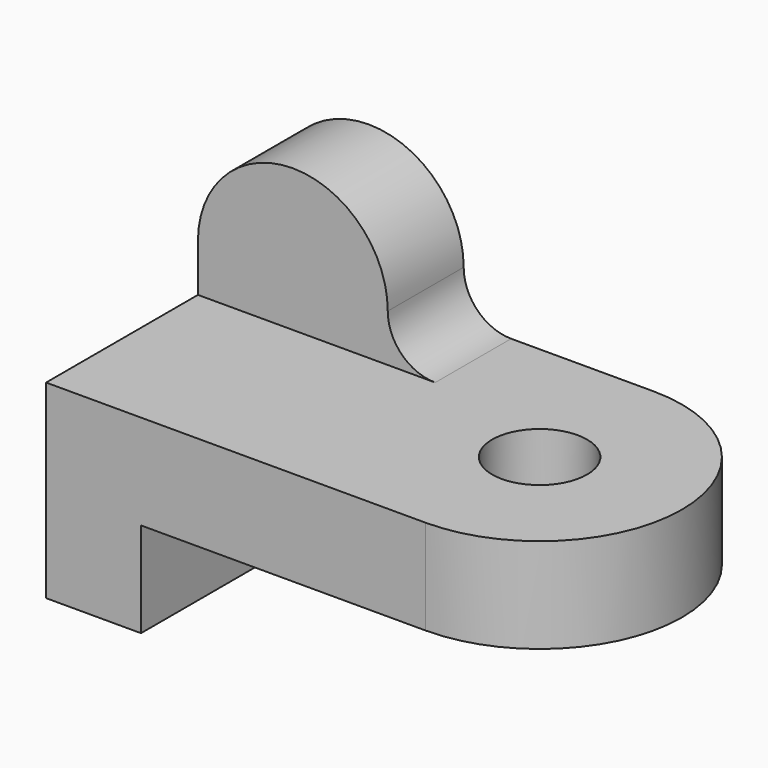
from build123d import *

# Parameters (mm, degrees)
F0_R     = 6.35
F0_W     = 12.7
F0_H     = 25.4
F0_H_2   = 12.7
F1_DEPTH = 12.7
F2_DEPTH = 12.7
F3_DEPTH = 19.05
F4_DEPTH = 12.7
F6_DEPTH = 12.7
F7_R     = 6.34999


# Not quite as in the source:
# - a fillet or chamfer is up to 0.001 mm smaller than in the source, because OpenCascade refuses the exact size


with BuildPart() as f1:
    # F0 (on Top) → F1 (new body)
    with BuildSketch(Plane.XY):
        with BuildLine():
            ThreePointArc((0, -17.2810847643), (19.05, 1.7689152357), (0, 20.8189152357))
            Line((0, 20.8189152357), (-25.4, 20.8189152357))
            Line((-25.4, 20.8189152357), (-25.4, 8.1189152357))
            Line((-25.4, 8.1189152357), (-38.1, 8.1189152357))
            Line((-38.1, 8.1189152357), (-38.1, -17.2810847643))
            Line((-38.1, -17.2810847643), (0, -17.2810847643))
        make_face()
        with Locations((0, 1.7689152357)):
            Circle(F0_R, mode=Mode.SUBTRACT)
        with Locations((-44.45, -4.5810847643)):
            Rectangle(F0_W, F0_H)
        with Locations((-44.45, 14.4689152357)):
            Rectangle(F0_W, F0_H_2)
        with Locations((-31.75, 14.4689152357)):
            Rectangle(F0_W, F0_H_2)
    extrude(amount=F1_DEPTH)

    # F0 (on Top) → F2 (join)
    with BuildSketch(Plane.XY):
        with Locations((-44.45, -4.5810847643)):
            Rectangle(F0_W, F0_H)
        with Locations((-44.45, 14.4689152357)):
            Rectangle(F0_W, F0_H_2)
    extrude(amount=-F2_DEPTH)

    # F0 (on Top) → F3 (join)
    with BuildSketch(Plane.XY):
        with Locations((-31.75, 14.4689152357)):
            Rectangle(F0_W, F0_H_2)
    extrude(amount=F3_DEPTH)

    # F4 (add): a face of the model
    f4_faces = [f1.faces().sort_by_distance(p)[0] for p in [
        (-38.1, 14.4689152357, 15.875),
    ]]
    extrude(f4_faces, amount=F4_DEPTH)

    # F5 (on face) → F6 (join)
    with BuildSketch(Plane.XZ.offset(-8.1189152357)):
        with BuildLine():
            Line((-50.8, 19.05), (-25.4, 19.05))
            ThreePointArc((-25.4, 19.05), (-38.1, 31.75), (-50.8, 19.05))
        make_face()
    extrude(amount=-F6_DEPTH)

    # F7 (radius 6.35 in the source; OpenCascade refuses exactly that, so slightly less here)
    f7_edges = [f1.edges().sort_by_distance(p)[0] for p in [
        (-25.4, 14.468915, 12.7),
    ]]
    fillet(f7_edges, radius=F7_R)


solid = f1.part
